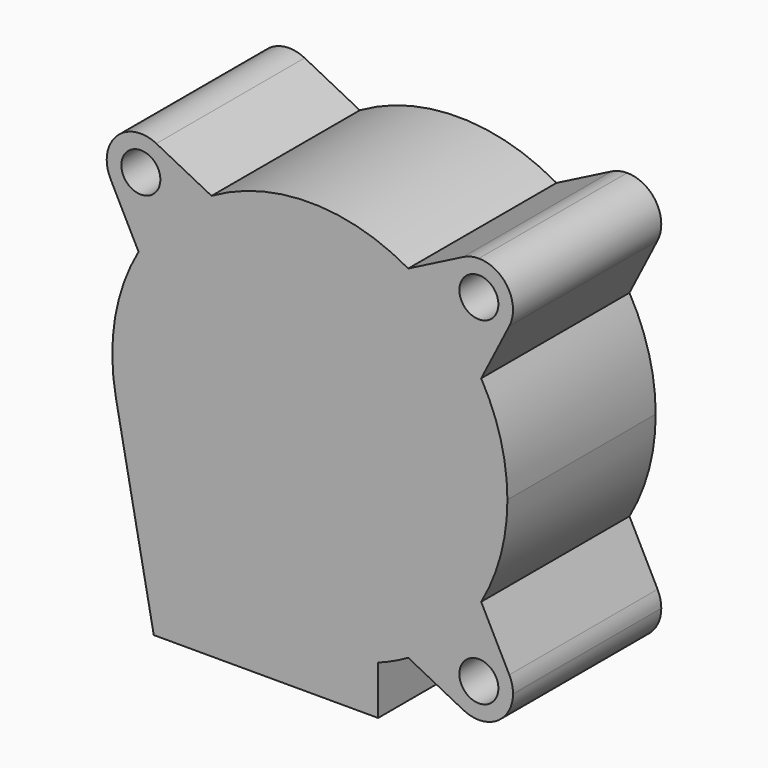
from build123d import *

# Parameters (mm, degrees)
F4_DEPTH        = 19
F5_T            = -2.5
F3_R            = 2
F6_DEPTH        = 19
F6_COPIES_COUNT = 3
F6_COPIES_ANGLE = 180


# Not quite as in the source:
# - a pattern or mirror of a feature is missing from the dataset's text; its kind, count and spacing are read off the source's solid


with BuildPart() as f1:
    # F0 (on Top) → F1 (revolve)
    with BuildSketch(Plane.XY):
        with BuildLine():
            Line((2.5, 8.5), (2.5, -3.5))
            Line((2.5, -3.5), (6, -3.5))
            Line((6, -3.5), (6, -2))
            ThreePointArc((6, -2), (5, 0), (6, 2))
            Line((6, 2), (6, 8.5))
            Line((6, 8.5), (2.5, 8.5))
        make_face()
    revolve(axis=Axis((0, 9.24498985, 0), (0, 1, 0)))


with BuildPart() as f4:
    # F3 (on Front) → F4 (new body)
    with BuildSketch(Plane.XZ):
        with BuildLine():
            ThreePointArc((7, -19.0016446657), (-9.9524559943, -17.6355073554), (-19.8845949623, -3.8295408585))
            Line((-19.8845949623, -3.8295408585), (-16, -24))
            Line((-16, -24), (7, -24))
            Line((7, -24), (7, -19.0016446657))
        make_face()
        with BuildLine():
            ThreePointArc((17.5620061533, -10.0815891541), (19.566465248, -5.2168896574), (20.25, 0))
            ThreePointArc((20.25, 0), (-1.9234671838, 20.1584417551), (-19.8845949623, -3.8295408585))
            ThreePointArc((-19.8845949623, -3.8295408585), (-9.9524559943, -17.6355073554), (7, -19.0016446657))
            ThreePointArc((7, -19.0016446657), (8.5710741316, -18.3466396986), (10.0815891541, -17.5620061533))
            ThreePointArc((10.0815891541, -17.5620061533), (14.318912319, -14.318912319), (17.5620061533, -10.0815891541))
        make_face()
    extrude(amount=F4_DEPTH)

    # F5
    f5_openings = [f4.faces().sort_by_distance(p)[0] for p in [
        (-4.5, -9.5, -24),
    ]]
    offset(amount=F5_T, openings=f5_openings, kind=Kind.INTERSECTION)

    # F3 (on Front) → F6 (join, through all)
    with BuildSketch(Plane.XZ):
        with BuildLine():
            Line((20.4426389737, -15.73514939), (17.5620061533, -10.0815891541))
            ThreePointArc((17.5620061533, -10.0815891541), (14.318912319, -14.318912319), (10.0815891541, -17.5620061533))
            Line((10.0815891541, -17.5620061533), (15.73514939, -20.4426389737))
            ThreePointArc((15.73514939, -20.4426389737), (14.8492424049, -14.8492424049), (20.4426389737, -15.73514939))
        make_face()
        with BuildLine():
            ThreePointArc((20.8241161391, -17.3241161391), (20.7274108605, -16.5070573656), (20.4426389737, -15.73514939))
            ThreePointArc((20.4426389737, -15.73514939), (14.8492424049, -14.8492424049), (15.73514939, -20.4426389737))
            ThreePointArc((15.73514939, -20.4426389737), (19.1528611156, -20.3083567143), (20.8241161391, -17.3241161391))
        make_face()
        with Locations((17.3241161391, -17.3241161391)):
            Circle(F3_R, mode=Mode.SUBTRACT)
    f6 = extrude(amount=F6_DEPTH)

    # F6_copies: F6 ×3 about axis
    f6_copies_axis = Axis((0, 0, 0), (0, -1, 0))
    for i in range(1, F6_COPIES_COUNT):
        add(f6.rotate(f6_copies_axis, i * F6_COPIES_ANGLE / (F6_COPIES_COUNT - 1)))


solid = Compound([f1.part, f4.part])
